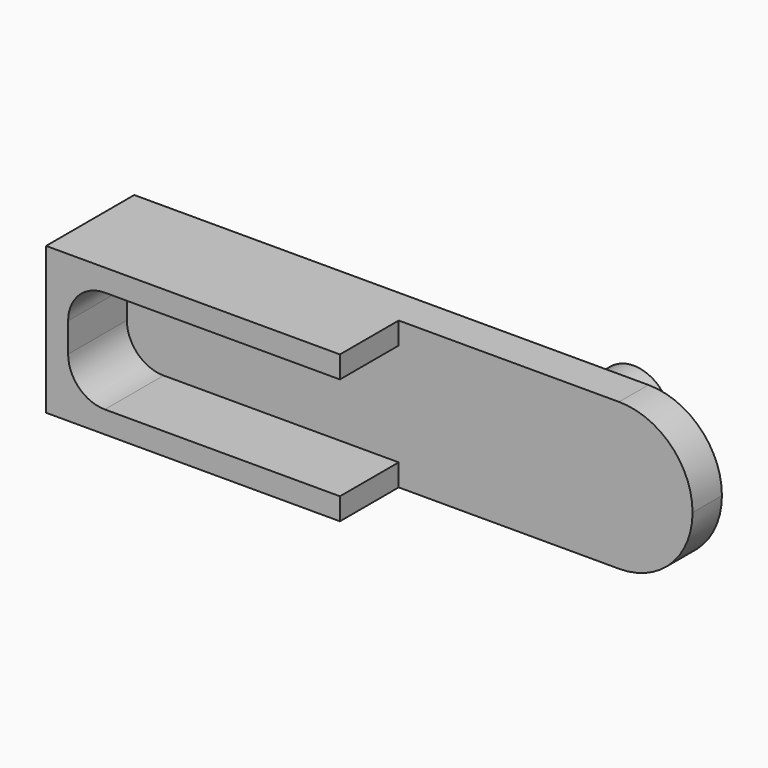
from build123d import *

# Parameters (mm, degrees)
F0_W     = 50.8
F0_H     = 12.7
F1_DEPTH = 3.175
F2_R     = 3.175
F3_DEPTH = 6.35
F5_DEPTH = 6.35
F6_R     = 3.175
F7_R     = 6.34999


# Not quite as in the source:
# - a fillet or chamfer is up to 0.001 mm smaller than in the source, because OpenCascade refuses the exact size


with BuildPart() as f1:
    # F0 (on Front) → F1 (new body)
    with BuildSketch(Plane.XZ):
        with Locations((1.988414675, -12.0237477115)):
            Rectangle(F0_W, F0_H)
    extrude(amount=F1_DEPTH)

    # F2 (on face) → F3 (join)
    with BuildSketch(Plane(origin=(0, 0, 0), x_dir=(-1, 0, 0), z_dir=(0, 1, 0))):
        with Locations((-14.688414675, -12.0237477115)):
            Circle(F2_R)
    extrude(amount=F3_DEPTH)

    # F4 (on face) → F5 (join)
    with BuildSketch(Plane.XZ.offset(3.175)):
        Polygon((1.988414675, -5.6737477115), (-23.411585325, -5.6737477115), (-23.411585325, -18.3737477115), (1.988414675, -18.3737477115), (1.988414675, -16.4687477115), (-21.506585325, -16.4687477115), (-21.506585325, -7.5787477115), (1.988414675, -7.5787477115), align=None)
    extrude(amount=F5_DEPTH)

    # F6
    f6_edges = [f1.edges().sort_by_distance(p)[0] for p in [
        (-21.506585, -6.35, -7.578748),
        (-21.506585, -6.35, -16.468748),
    ]]
    fillet(f6_edges, radius=F6_R)

    # F7 (radius 6.35 in the source; OpenCascade refuses exactly that, so slightly less here)
    f7_edges = [f1.edges().sort_by_distance(p)[0] for p in [
        (27.388415, -1.5875, -5.673748),
        (27.388415, -1.5875, -18.373748),
    ]]
    fillet(f7_edges, radius=F7_R)


solid = f1.part
